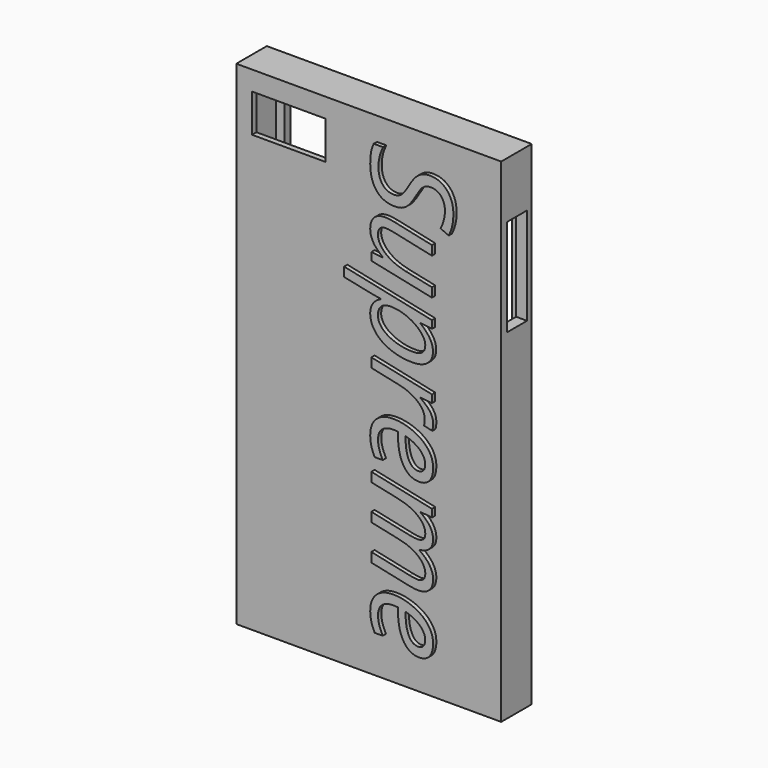
from build123d import *

# Parameters (mm, degrees)
F0_W         = 82.4865
F0_H         = 153.6065
F0_W_2       = 22.86
F0_H_2       = 11.851914227
F2_DEPTH     = 11.8745
F1_TEXT_SIZE = 35.2777777778
F3_DEPTH     = 1.27
F5_W         = 76.2
F5_H         = 148.59
F6_DEPTH     = 10.16
F7_W         = 70.8706876242
F7_H         = 2.5495670867
F8_DEPTH     = 2.54
F8_TAPER     = 3
F9_W         = 63.9890395105
F9_H         = 6.5411017276
F10_DEPTH    = 127
F11_W        = 7.8073232435
F11_H        = 30.2533730865
F12_DEPTH    = 101.6


# Not quite as in the source:
# - Text() gives the source's letters only with a copy of the font that has no kerning and outlines rounded to 1/6400 em; it was checked with that copy


with BuildPart() as f2:
    # F0 (on Front) → F2 (new body)
    with BuildSketch(Plane.XZ):
        with Locations((-4.1093219483, -3.8867425174)):
            Rectangle(F0_W, F0_H)
        with Locations((-29.0071740296, 60.953464359)):
            Rectangle(F0_W_2, F0_H_2, mode=Mode.SUBTRACT)
    extrude(amount=-F2_DEPTH)

    # F1 (on Front) → F3 (join)
    with BuildSketch(Plane.XZ):
        with Locations(Location((-2.2859999444, 66.4048695471), (0, 0, -90))):
            Text('Supreme', F1_TEXT_SIZE, font='Open Sans', font_style=FontStyle.ITALIC, text_align=(TextAlign.LEFT, TextAlign.BOTTOM))
    extrude(amount=F3_DEPTH)

    # F5 (on offset) → F6 (cut)
    with BuildSketch(Plane.XZ.offset(-11.8745)):
        with Locations((-4.3659678671, -3.6440938711)):
            Rectangle(F5_W, F5_H)
    extrude(amount=F6_DEPTH, mode=Mode.SUBTRACT)

    # F9 (on Top) → F10 (cut)
    with BuildSketch(Plane.XY):
        with Locations((-2.7680639178, 6.520740455)):
            Rectangle(F9_W, F9_H)
    extrude(amount=-F10_DEPTH, mode=Mode.SUBTRACT)

    # F11 (on Right) → F12 (cut)
    with BuildSketch(Plane.YZ):
        with Locations((6.1482668389, 40.3049103916)):
            Rectangle(F11_W, F11_H)
    extrude(amount=F12_DEPTH, mode=Mode.SUBTRACT)


with BuildPart() as f8:
    # F7 (on offset) → F8 (new body)
    with BuildSketch(Plane.XZ.offset(-11.8745)):
        Polygon((33.7340321329, -77.9390938711), (33.7340321329, 70.6509061289), (30.9528460705, 70.6509061289), (30.9528460705, 68.1160017848), (30.9528460705, -75.3895267844), (30.9528460705, -77.9390938711), align=None)
        Polygon((30.9528460705, 68.1160017848), (30.9528460705, 70.6509061289), (-42.4659678671, 70.6509061289), (-42.4659678671, 68.1160017848), (-39.9178415537, 68.1160017848), align=None)
        with Locations((-4.4824977416, -76.6643103278)):
            Rectangle(F7_W, F7_H)
        Polygon((-39.9178415537, -75.3895267844), (-39.9178415537, 68.1160017848), (-42.4659678671, 68.1160017848), (-42.4659678671, -77.9390938711), (-39.9178415537, -77.9390938711), align=None)
    extrude(amount=-F8_DEPTH, taper=F8_TAPER)


solid = Compound([f2.part, f8.part])
